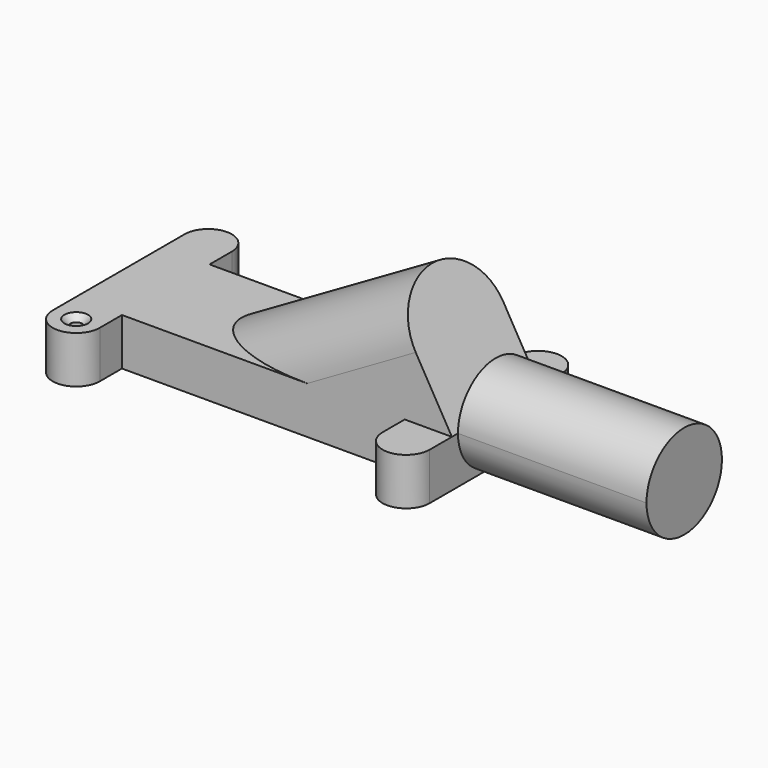
from build123d import *

# Parameters (mm, degrees)
F1_DEPTH        = 25.4
F6_DEPTH        = 101.6
F10_D           = 6.35
F10_CSINK_D     = 12.7
F10_CSINK_ANGLE = 90


with BuildPart() as f1:
    # F0 (on Top) → F1 (new body)
    with BuildSketch(Plane.XY):
        with BuildLine():
            Line((0, -59.0296), (0, 0))
            Line((0, 0), (-76.2, 0))
            Line((-76.2, 0), (-76.2, 14.9352))
            ThreePointArc((-76.2, 14.9352), (-88.9, 27.6352), (-101.6, 14.9352))
            Line((-101.6, 14.9352), (-101.6, -73.9648))
            ThreePointArc((-101.6, -73.9648), (-88.9, -86.6648), (-76.2, -73.9648))
            Line((-76.2, -73.9648), (-76.2, -59.0296))
            Line((-76.2, -59.0296), (0, -59.0296))
        make_face()
        with BuildLine():
            Line((76.2, 0), (0, 0))
            Line((0, 0), (0, -59.0296))
            Line((0, -59.0296), (76.2, -59.0296))
            Line((76.2, -59.0296), (76.2, -73.9648))
            ThreePointArc((76.2, -73.9648), (88.9, -86.6648), (101.6, -73.9648))
            Line((101.6, -73.9648), (101.6, 14.9352))
            ThreePointArc((101.6, 14.9352), (88.9, 27.6352), (76.2, 14.9352))
            Line((76.2, 14.9352), (76.2, 0))
        make_face()
    extrude(amount=F1_DEPTH)

    # F3 (on face) → F4 (join, up to the next surface of F1)
    with BuildSketch(Plane(origin=(87.1985226281, 0, 50.3440905122), x_dir=(0, 1, 0), z_dir=(0.8660254038, 0, 0.5))):
        with BuildLine():
            Line((-59.0296, 10.1618718698), (-59.0296, -28.8029547439))
            Line((-59.0296, -28.8029547439), (0, -28.8029547439))
            Line((0, -28.8029547439), (0, 10.1618718698))
            ThreePointArc((0, 10.1618718698), (-29.5148, 39.6766718698), (-59.0296, 10.1618718698))
        make_face()
    extrude(until=Until.NEXT, dir=(-0.8660254038, 0, -0.5))

    # F5 (on face) → F6 (join)
    with BuildSketch(Plane.YZ.offset(101.6)):
        with BuildLine():
            Line((-54.9148, 25.4), (-4.1148, 25.4))
            ThreePointArc((-4.1148, 25.4), (-29.5148, 50.8), (-54.9148, 25.4))
        make_face()
        with BuildLine():
            ThreePointArc((-29.5148, 0), (-11.5542877579, 7.4394877579), (-4.1148, 25.4))
            Line((-4.1148, 25.4), (-54.9148, 25.4))
            ThreePointArc((-54.9148, 25.4), (-47.4753122421, 7.4394877579), (-29.5148, 0))
        make_face()
    extrude(amount=F6_DEPTH)

    # F10 (through all)
    with Locations(Plane.XY.offset(25.4)):
        with Locations((-88.9, -73.9648)):
            CounterSinkHole(F10_D / 2, F10_CSINK_D / 2, counter_sink_angle=F10_CSINK_ANGLE)


solid = f1.part
